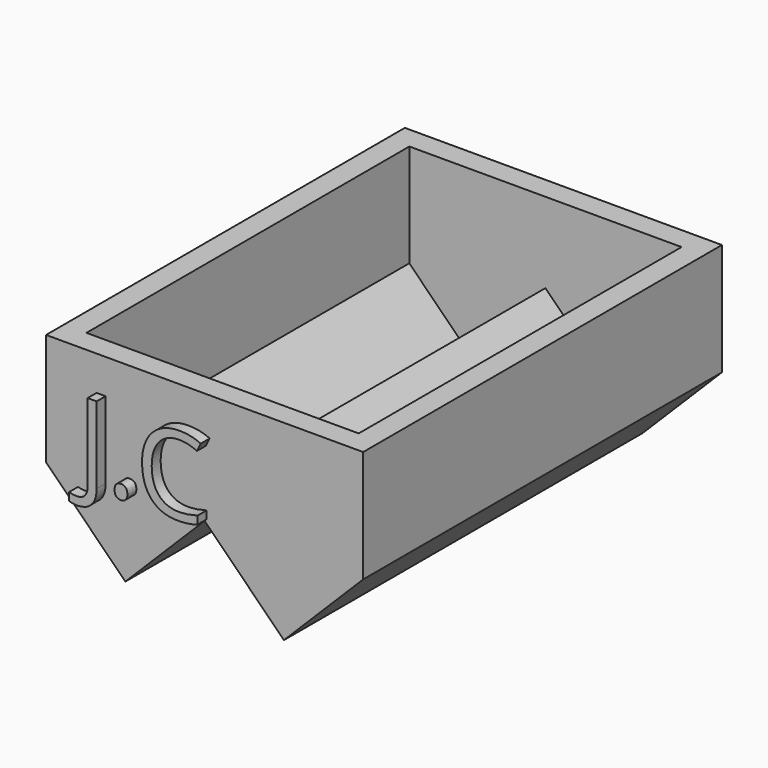
from build123d import *

# Parameters (mm, degrees)
F1_DEPTH     = 50.8
F2_T         = -2.54
F3_TEXT_SIZE = 12.3000949518
F4_DEPTH     = 1.27


# Not quite as in the source:
# - Text() gives the source's letters only with a copy of the font that has no kerning and outlines rounded to 1/6400 em; it was checked with that copy


with BuildPart() as f1:
    # F0 (on Front) → F1 (new body)
    with BuildSketch(Plane.XZ):
        Polygon((-6.3743383161, 17.7387978554), (-42.2953628004, 17.7387978554), (-42.2953628004, 5.0387978554), (-33.3151066793, -3.9414582657), (-24.3348505582, 5.0387978554), (-15.3545944372, -3.9414582657), (-6.3743383161, 5.0387978554), align=None)
    extrude(amount=F1_DEPTH)

    # F2
    f2_openings = [f1.faces().sort_by_distance(p)[0] for p in [
        (-24.334851, -25.4, 17.738798),
    ]]
    offset(amount=F2_T, openings=f2_openings, kind=Kind.INTERSECTION)

    # F3 (on face) → F4 (join)
    with BuildSketch(Plane.XZ.offset(50.8)):
        with Locations((-37.714637816, 5.0387978554)):
            Text('J.C', F3_TEXT_SIZE, font='Open Sans', text_align=(TextAlign.LEFT, TextAlign.BOTTOM))
    extrude(amount=F4_DEPTH)


solid = f1.part
